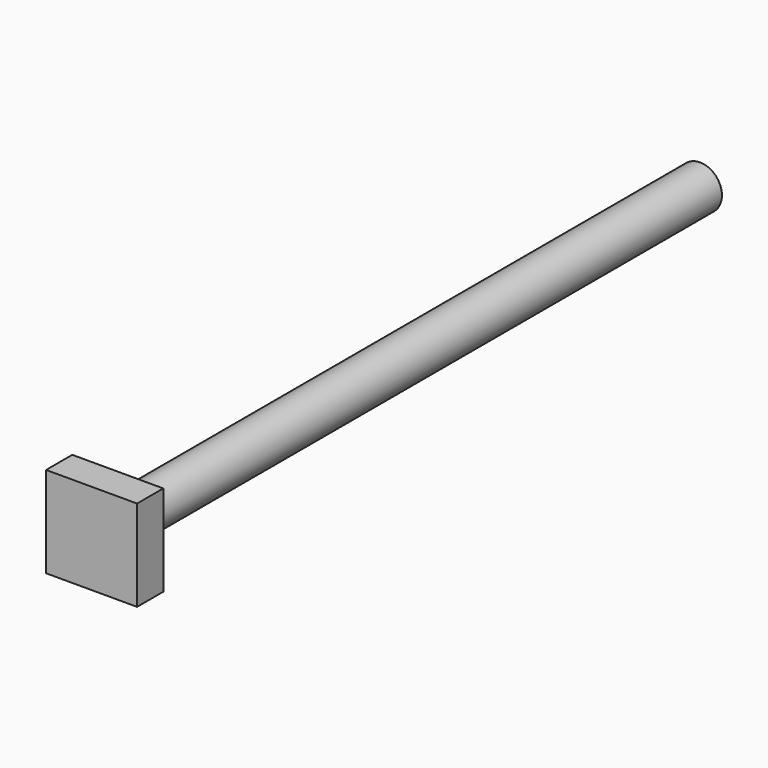
from build123d import *

# Parameters (mm, degrees)
F0_R     = 6
F1_DEPTH = 200
F2_R     = 6
F0_W     = 25
F0_H     = 25
F3_DEPTH = 9


with BuildPart() as f1:
    # F0 (on Front) → F1 (new body)
    with BuildSketch(Plane.XZ):
        Circle(F0_R)
    extrude(amount=-F1_DEPTH)

    # F2 (on face) + F0 (on Front) → F3 (join)
    with BuildSketch(Plane.XZ):
        Circle(F2_R)
    with BuildSketch(Plane.XZ):
        Rectangle(F0_W, F0_H)
        Circle(F0_R, mode=Mode.SUBTRACT)
    extrude(amount=F3_DEPTH)


solid = f1.part
